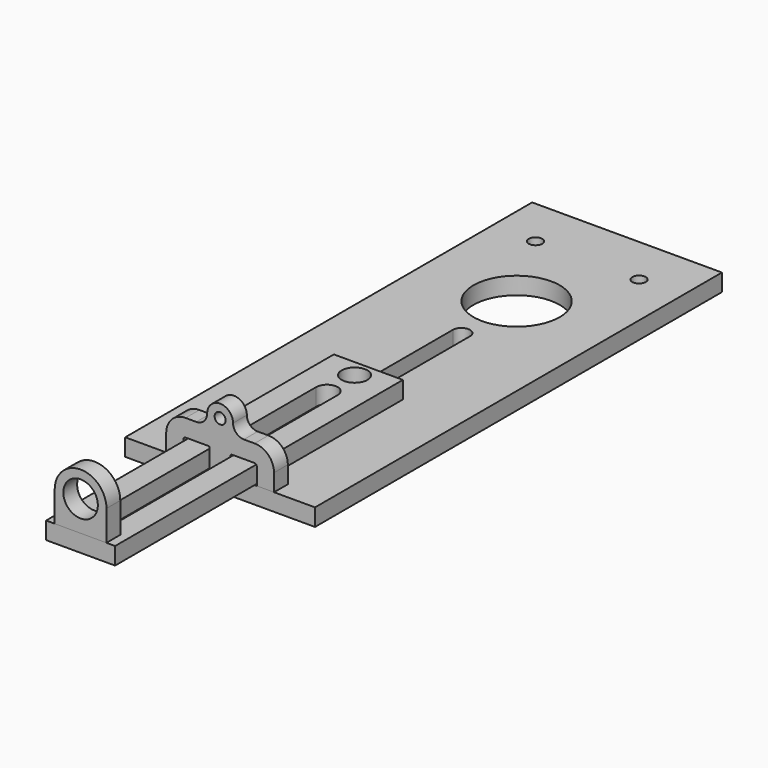
from build123d import *

# Parameters (mm, degrees)
F2_W            = 69.85
F2_H            = 187.2107
F2_R            = 1.4732
F2_R_2          = 2.15265
F2_R_3          = 15.875
F3_DEPTH        = 6.35
F4_W            = 25.4
F4_H            = 132.3975
F4_R            = 1.4732
F4_R_2          = 4.7625
F5_DEPTH        = 6.35
F6_R            = 2.0193
F7_DEPTH        = 6.35
F8_R            = 6.35
F9_DEPTH        = 6.35
F10_R           = 1.4732
F11_DEPTH       = 6.351
F12_D           = 4.9784
F12_CSINK_D     = 10.4394
F12_CSINK_ANGLE = 82
F13_D           = 2.9464
F13_CSINK_D     = 6.477
F13_CSINK_ANGLE = 82
F14_DEPTH       = 12.7
F15_DEPTH       = 19.05


# Not quite as in the source:
# - a variable given as a bare number and used for a length is read in inches; the dataset says mm whatever the document's units were


with BuildPart() as f3:
    # F2 (on Top) → F3 (new body)
    with BuildSketch(Plane.XY):
        Rectangle(F2_W, F2_H)
        with Locations((0, -90.43035)):
            Circle(F2_R, mode=Mode.SUBTRACT)
        with Locations((0, -74.66965)):
            Circle(F2_R_2, mode=Mode.SUBTRACT)
        with BuildLine():
            ThreePointArc((-3.175, 17.40535), (0, 20.58035), (3.175, 17.40535))
            Line((3.175, 17.40535), (3.175, -58.79465))
            ThreePointArc((3.175, -58.79465), (0, -61.96965), (-3.175, -58.79465))
            Line((-3.175, -58.79465), (-3.175, 17.40535))
        make_face(mode=Mode.SUBTRACT)
        with Locations((-19.05, 75.31735)):
            Circle(F2_R_2, mode=Mode.SUBTRACT)
        with Locations((0, 42.80535)):
            Circle(F2_R_3, mode=Mode.SUBTRACT)
        with Locations((19.05, 75.31735)):
            Circle(F2_R_2, mode=Mode.SUBTRACT)
    extrude(amount=F3_DEPTH)

    # F10 (on face) → F11 (cut, through all)
    with BuildSketch(Plane(origin=(0, 0, 6.35), x_dir=(1, 0, 0), z_dir=(0, 0, -1))):
        with Locations((-16.66875, 90.43035)):
            Circle(F10_R)
        with Locations((16.66875, 90.43035)):
            Circle(F10_R)
    extrude(amount=F11_DEPTH, mode=Mode.SUBTRACT)

    # F12 (through all)
    with Locations(Plane(origin=(0, 0, 0), x_dir=(1, 0, 0), z_dir=(0, 0, -1))):
        with Locations((19.05, -75.31735), (-19.05, -75.31735), (0, 74.66965)):
            CounterSinkHole(F12_D / 2, F12_CSINK_D / 2, counter_sink_angle=F12_CSINK_ANGLE)

    # F13 (through all)
    with Locations(Plane(origin=(0, 0, 0), x_dir=(1, 0, 0), z_dir=(0, 0, -1))):
        with Locations((0, 90.43035)):
            CounterSinkHole(F13_D / 2, F13_CSINK_D / 2, counter_sink_angle=F13_CSINK_ANGLE)


with BuildPart() as f5:
    # F4 (on face) → F5 (new body)
    with BuildSketch(Plane.XY.offset(6.35)):
        with Locations((0, -91.59875)):
            Rectangle(F4_W, F4_H)
        with Locations((-6.35, -154.6225)):
            Circle(F4_R, mode=Mode.SUBTRACT)
        with BuildLine():
            ThreePointArc((-3.96875, -44.45), (0, -40.48125), (3.96875, -44.45))
            Line((3.96875, -44.45), (3.96875, -143.51))
            ThreePointArc((3.96875, -143.51), (0, -147.47875), (-3.96875, -143.51))
            Line((-3.96875, -143.51), (-3.96875, -44.45))
        make_face(mode=Mode.SUBTRACT)
        with Locations((6.35, -154.6225)):
            Circle(F4_R, mode=Mode.SUBTRACT)
        with Locations((0, -31.75)):
            Circle(F4_R_2, mode=Mode.SUBTRACT)
    extrude(amount=F5_DEPTH)


with BuildPart() as f7:
    # F6 (on face) → F7 (new body)
    with BuildSketch(Plane.XZ.offset(93.60535)):
        with BuildLine():
            ThreePointArc((8.763, 19.84375), (5.9342193219, 21.0154693219), (4.7625, 23.84425))
            ThreePointArc((4.7625, 23.84425), (0, 28.60675), (-4.7625, 23.84425))
            ThreePointArc((-4.7625, 23.84425), (-5.9342193219, 21.0154693219), (-8.763, 19.84375))
            Line((-8.763, 19.84375), (-12.7, 19.84375))
            ThreePointArc((-12.7, 19.84375), (-17.7513940681, 17.7513940681), (-19.84375, 12.7))
            Line((-19.84375, 12.7), (-19.84375, 6.35))
            Line((-19.84375, 6.35), (-13.49375, 6.35))
            Line((-13.49375, 6.35), (-13.49375, 12.7))
            ThreePointArc((-13.49375, 12.7), (-13.2612660076, 13.2612660076), (-12.7, 13.49375))
            Line((-12.7, 13.49375), (-4.289425, 13.49375))
            ThreePointArc((-4.289425, 13.49375), (-4.0087919962, 13.3775080038), (-3.89255, 13.096875))
            Line((-3.89255, 13.096875), (-3.89255, 6.35))
            Line((-3.89255, 6.35), (0, 6.35))
            Line((0, 6.35), (3.89255, 6.35))
            Line((3.89255, 6.35), (3.89255, 13.096875))
            ThreePointArc((3.89255, 13.096875), (4.0087919962, 13.3775080038), (4.289425, 13.49375))
            Line((4.289425, 13.49375), (12.7, 13.49375))
            ThreePointArc((12.7, 13.49375), (13.2612660076, 13.2612660076), (13.49375, 12.7))
            Line((13.49375, 12.7), (13.49375, 6.35))
            Line((13.49375, 6.35), (19.84375, 6.35))
            Line((19.84375, 6.35), (19.84375, 12.7))
            ThreePointArc((19.84375, 12.7), (17.7513940681, 17.7513940681), (12.7, 19.84375))
            Line((12.7, 19.84375), (8.763, 19.84375))
        make_face()
        with Locations((0, 23.84425)):
            Circle(F6_R, mode=Mode.SUBTRACT)
    extrude(amount=-F7_DEPTH)

    # F2 (on Top) → F15 (cut)
    with BuildSketch(Plane.XY):
        with Locations((0, -90.43035)):
            Circle(F2_R)
    extrude(amount=F15_DEPTH, mode=Mode.SUBTRACT)


with BuildPart() as f9:
    # F8 (on face) → F9 (new body)
    with BuildSketch(Plane.XZ.offset(157.7975)):
        with BuildLine():
            Line((-9.525, 23.84425), (-9.525, 12.7))
            Line((-9.525, 12.7), (9.525, 12.7))
            Line((9.525, 12.7), (9.525, 23.84425))
            ThreePointArc((9.525, 23.84425), (0, 33.36925), (-9.525, 23.84425))
        make_face()
        with Locations((0, 23.84425)):
            Circle(F8_R, mode=Mode.SUBTRACT)
    extrude(amount=-F9_DEPTH)

    # F4 (on face) → F14 (cut)
    with BuildSketch(Plane.XY.offset(6.35)):
        with Locations((6.35, -154.6225)):
            Circle(F4_R)
        with Locations((-6.35, -154.6225)):
            Circle(F4_R)
    extrude(amount=F14_DEPTH, mode=Mode.SUBTRACT)


solid = Compound([f3.part, f5.part, f7.part, f9.part])
